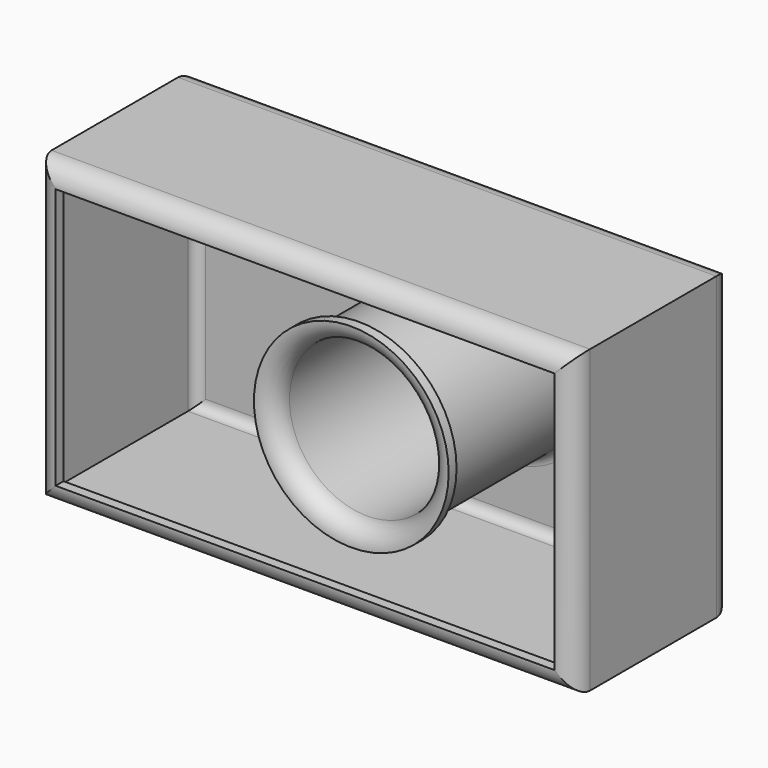
from build123d import *

# Parameters (mm, degrees)
F0_W     = 138.4936049581
F0_H     = 77.3329418153
F0_R     = 19.9688682615
F1_DEPTH = 50.8
F2_R     = 5.08
F3_R     = 5.08
F4_T     = -2.54


# Not quite as in the source:
# - a shell that OpenCascade refuses in one call is made with other operations: the cavity is built on its own and cut out


with BuildPart() as f1:
    # F0 (on Front) → F1 (new body)
    with BuildSketch(Plane.XZ):
        with Locations((-2.6111938059, 14.1139933839)):
            Rectangle(F0_W, F0_H)
        with Locations((9.2974901199, 16.3193047047)):
            Circle(F0_R, mode=Mode.SUBTRACT)
    extrude(amount=F1_DEPTH)

    # F2
    f2_edges = [f1.edges().sort_by_distance(p)[0] for p in [
        (66.635609, 0, 14.113993),
        (-2.611194, 0, 52.780464),
        (-71.857996, 0, 14.113993),
        (-2.611194, 0, -24.552478),
        (-10.671378, 0, 16.319305),
        (-10.671378, -50.8, 16.319305),
    ]]
    fillet(f2_edges, radius=F2_R)

    # F3
    f3_edges = [f1.edges().sort_by_distance(p)[0] for p in [
        (-2.611194, -50.8, -24.552478),
        (-71.857996, -50.8, 14.113993),
        (-2.611194, -50.8, 52.780464),
        (66.635609, -50.8, 14.113993),
    ]]
    fillet(f3_edges, radius=F3_R)

    # F4: a shell. OpenCascade refuses it in one call, so the cavity is built on its own and cut out:
    # the body offset inwards by the wall thickness, plus a prism from it out through each open face.
    f4_core = offset(f1.part, amount=F4_T, mode=Mode.PRIVATE)
    f4_exits = [f4_core.faces().sort_by_distance(p)[0] for p in [
        (-2.611194, -48.26, -18.023971),
    ]]
    add(f4_core, mode=Mode.SUBTRACT)
    extrude(f4_exits, amount=-F4_T, mode=Mode.SUBTRACT)


solid = f1.part
